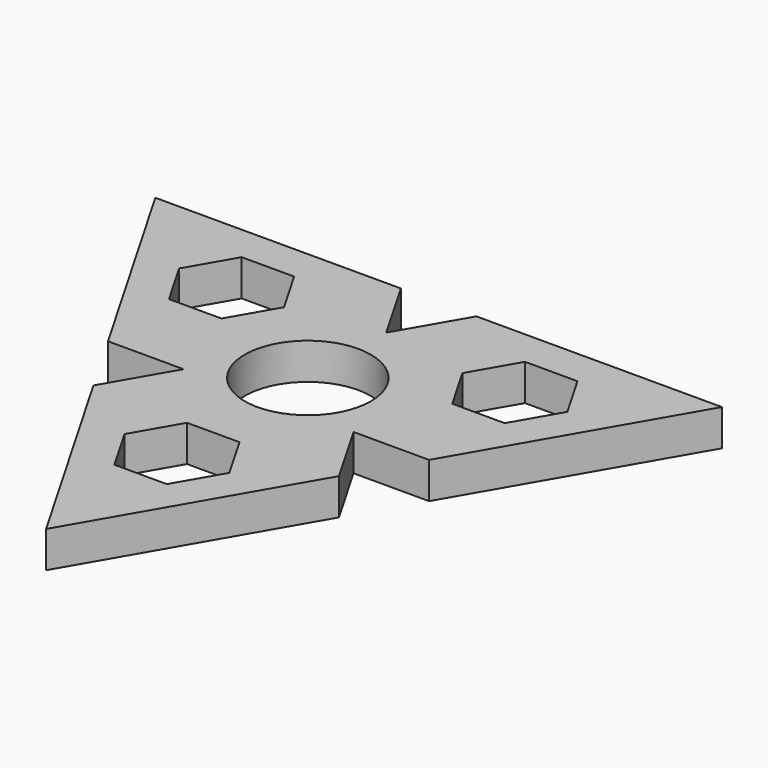
from build123d import *

# Parameters (mm, degrees)
F0_R     = 11.0236
F1_DEPTH = 6.35
F3_DEPTH = 6.35


with BuildPart() as f1:
    # F0 (on Top) → F1 (new body)
    with BuildSketch(Plane.XY):
        Polygon((0, -57.15), (24.7466759131, -14.2875), (-24.7466759131, -14.2875), align=None)
        Polygon((-4.5827177617, -36.5125), (-9.1654355234, -28.575), (-4.5827177617, -20.6375), (4.5827177617, -20.6375), (9.1654355234, -28.575), (4.5827177617, -36.5125), align=None, mode=Mode.SUBTRACT)
        Polygon((-24.7466759131, -14.2875), (24.7466759131, -14.2875), (0, 28.575), align=None)
        Circle(F0_R, mode=Mode.SUBTRACT)
        Polygon((0, 28.575), (24.7466759131, -14.2875), (49.4933518263, 28.575), align=None)
        Polygon((33.9121114365, 14.2875), (29.3293936748, 6.35), (20.1639581514, 6.35), (15.5812403898, 14.2875), (20.1639581514, 22.225), (29.3293936748, 22.225), align=None, mode=Mode.SUBTRACT)
        Polygon((-49.4933518263, 28.575), (-24.7466759131, -14.2875), (0, 28.575), align=None)
        Polygon((-20.1639581514, 22.225), (-15.5812403898, 14.2875), (-20.1639581514, 6.35), (-29.3293936748, 6.35), (-33.9121114365, 14.2875), (-29.3293936748, 22.225), align=None, mode=Mode.SUBTRACT)
    extrude(amount=F1_DEPTH)

    # F2 (on face) → F3 (cut)
    with BuildSketch(Plane.XY.offset(6.35)):
        Polygon((6.5991135768, 28.575), (-6.5991135768, 28.575), (0, 17.145), align=None)
        Polygon((-14.8480055479, -8.5725), (-28.0462327016, -8.5725), (-21.4471191247, -20.0025), align=None)
        Polygon((21.4471191247, -20.0025), (28.0462327016, -8.5725), (14.8480055479, -8.5725), align=None)
    extrude(amount=-F3_DEPTH, mode=Mode.SUBTRACT)


solid = f1.part
